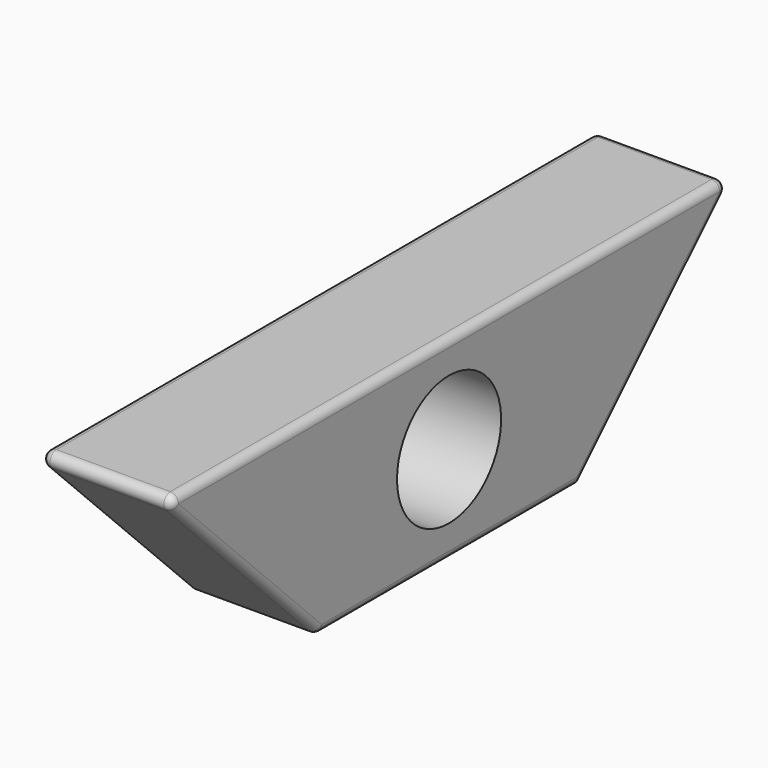
from build123d import *

# Parameters (mm, degrees)
F1_DEPTH = 50.8
F3_D     = 50.8
F4_R     = 3.175


# Not quite as in the source:
# - a feature of the source that left no trace in its solid (it failed there, or was rolled back) is left out


with BuildPart() as f1:
    # F0 (on Right) → F1 (new body)
    with BuildSketch(Plane.YZ):
        Polygon((208.5787526399, 38.1), (-70.8212473601, 38.1), (5.3787526399, -38.1), (132.3787526399, -38.1), align=None)
    extrude(amount=F1_DEPTH)

    # F3 (through all)
    with Locations(Plane(origin=(0, 0, 0), x_dir=(0, 1, 0), z_dir=(-1, 0, 0))):
        with Locations((68.8787526399, 0)):
            Hole(F3_D / 2)

    # F4
    f4_edges = [f1.edges().sort_by_distance(p)[0] for p in [
        (0, 68.878753, 38.1),
        (25.4, 5.378753, -38.1),
        (0, 68.878753, -38.1),
        (50.8, 68.878753, -38.1),
        (25.4, -70.821247, 38.1),
        (0, -32.721247, 0),
        (50.8, -32.721247, 0),
        (25.4, 208.578753, 38.1),
        (0, 170.478753, 0),
        (50.8, 170.478753, 0),
        (50.8, 68.878753, 38.1),
    ]]
    fillet(f4_edges, radius=F4_R)


solid = f1.part
